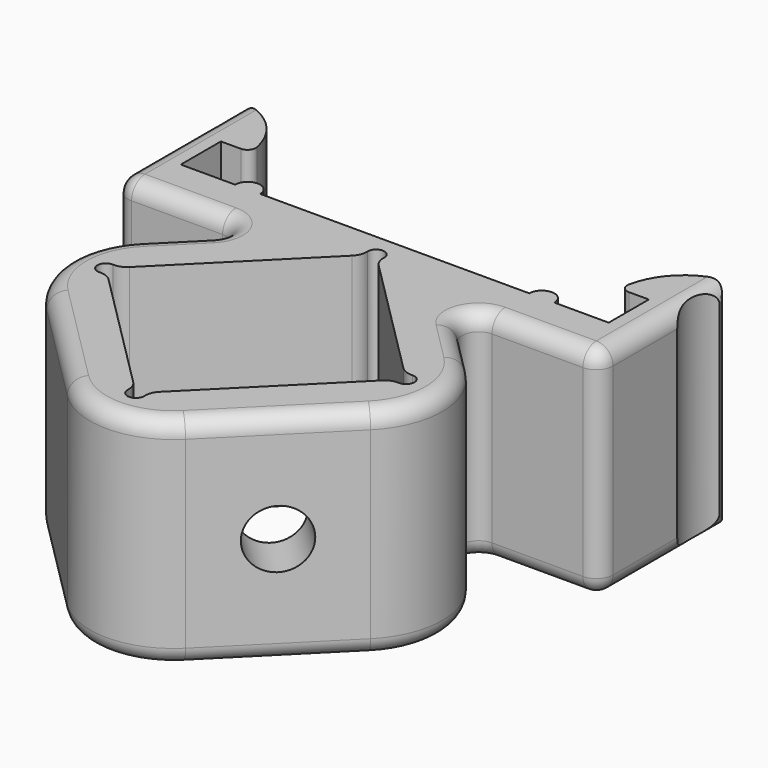
from build123d import *

# Parameters (mm, degrees)
F1_DEPTH  = 13
F4_DEPTH  = 13.001
F5_R      = 0.49999
F6_R      = 1
F7_R      = 5
F8_R      = 1
F9_R      = 0.5
F10_R     = 1
F11_R     = 1.75
F12_DEPTH = 15.6999998824


# Not quite as in the source:
# - a fillet or chamfer is up to 0.001 mm smaller than in the source, because OpenCascade refuses the exact size


with BuildPart() as f1:
    # F0 (on Top) → F1 (new body)
    with BuildSketch(Plane.XY):
        with BuildLine():
            ThreePointArc((-14.5, 1), (-14.2071067812, 0.2928932188), (-13.5, 0))
            Line((-13.5, 0), (-5.6426405208, 0))
            Line((-5.6426405208, 0), (-13.2228966419, -7.5802561211))
            Line((-13.2228966419, -7.5802561211), (0, -20.803152763))
            Line((0, -20.803152763), (13.2228966419, -7.5802561211))
            Line((13.2228966419, -7.5802561211), (5.6426405208, 0))
            Line((5.6426405208, 0), (13.5, 0))
            ThreePointArc((13.5, 0), (14.2071067812, 0.2928932188), (14.5, 1))
            Line((14.5, 1), (14.5, 9.5887489808))
            ThreePointArc((14.5, 9.5887489808), (12.0898455808, 8.3182698074), (11.05, 5.8))
            Line((11.05, 5.8), (12.8, 5.8))
            Line((12.8, 5.8), (12.8, 2.8))
            Line((12.8, 2.8), (9.55, 2.8))
            ThreePointArc((9.55, 2.8), (8.8, 3.55), (8.05, 2.8))
            Line((8.05, 2.8), (-8.05, 2.8))
            ThreePointArc((-8.05, 2.8), (-8.8, 3.55), (-9.55, 2.8))
            Line((-9.55, 2.8), (-12.8, 2.8))
            Line((-12.8, 2.8), (-12.8, 5.8))
            Line((-12.8, 5.8), (-11.05, 5.8))
            ThreePointArc((-11.05, 5.8), (-12.0898455808, 8.3182698074), (-14.5, 9.5887489808))
            Line((-14.5, 9.5887489808), (-14.5, 1))
        make_face()
        with BuildLine():
            Line((-8.6267027305, -7.2267027305), (-0.3535533906, 1.0464466094))
            ThreePointArc((-0.3535533906, 1.0464466094), (0, 1.9), (0.3535533906, 1.0464466094))
            Line((0.3535533906, 1.0464466094), (8.6267027305, -7.2267027305))
            ThreePointArc((8.6267027305, -7.2267027305), (9.4802561211, -7.5802561211), (8.6267027305, -7.9338095117))
            Line((8.6267027305, -7.9338095117), (0.3535533906, -16.2069588515))
            ThreePointArc((0.3535533906, -16.2069588515), (0, -17.0605122421), (-0.3535533906, -16.2069588515))
            Line((-0.3535533906, -16.2069588515), (-8.6267027305, -7.9338095117))
            ThreePointArc((-8.6267027305, -7.9338095117), (-9.4802561211, -7.5802561211), (-8.6267027305, -7.2267027305))
        make_face(mode=Mode.SUBTRACT)
    extrude(amount=F1_DEPTH)

    # F3 (on face) → F4 (cut, through all)
    with BuildSketch(Plane.XY.offset(13)):
        with BuildLine():
            ThreePointArc((-14.5, 5.8), (-14.0485078359, 7.3827532374), (-14.5, 8.9655064748))
            Line((-14.5, 8.9655064748), (-14.5, 5.8))
        make_face()
        with BuildLine():
            Line((14.5, 5.8), (14.5, 8.9655064748))
            ThreePointArc((14.5, 8.9655064748), (14.0485078359, 7.3827532374), (14.5, 5.8))
        make_face()
    extrude(amount=-F4_DEPTH, mode=Mode.SUBTRACT)

    # F5 (radius 0.5 in the source; OpenCascade refuses exactly that, so slightly less here)
    f5_edges = [f1.edges().sort_by_distance(p)[0] for p in [
        (-14.5, 9.588749, 6.5),
        (14.5, 9.588749, 6.5),
    ]]
    fillet(f5_edges, radius=F5_R)

    # F6
    f6_edges = [f1.edges().sort_by_distance(p)[0] for p in [
        (-5.642641, 0, 6.5),
        (5.642641, 0, 6.5),
    ]]
    fillet(f6_edges, radius=F6_R)

    # F7
    f7_edges = [f1.edges().sort_by_distance(p)[0] for p in [
        (-13.222897, -7.580256, 6.5),
        (0, -20.803153, 6.5),
        (13.222897, -7.580256, 6.5),
    ]]
    fillet(f7_edges, radius=F7_R)

    # F8
    f8_edges = [f1.edges().sort_by_distance(p)[0] for p in [
        (-6.611448, -14.191704, 13),
        (-6.611448, -14.191704, 0),
    ]]
    fillet(f8_edges, radius=F8_R)

    # F9
    f9_edges = [f1.edges().sort_by_distance(p)[0] for p in [
        (-11.05, 5.8, 6.5),
        (11.05, 5.8, 6.5),
    ]]
    fillet(f9_edges, radius=F9_R)

    # F10
    f10_edges = [f1.edges().sort_by_distance(p)[0] for p in [
        (-0.353553, 1.046447, 6.5),
        (0.353553, 1.046447, 6.5),
        (-8.626703, -7.226703, 6.5),
        (-8.626703, -7.93381, 6.5),
        (-0.353553, -16.206959, 6.5),
        (0.353553, -16.206959, 6.5),
        (8.626703, -7.226703, 6.5),
        (8.626703, -7.93381, 6.5),
    ]]
    fillet(f10_edges, radius=F10_R)

    # F11 (on face) → F12 (cut, through all)
    with BuildSketch(Plane(origin=(10.4015763815, -10.4015763815, 0), x_dir=(0.7071067812, 0.7071067812, 0), z_dir=(0.7071067812, -0.7071067812, 0))):
        with Locations((-5.3600505063, 6.5)):
            Circle(F11_R)
    extrude(amount=-F12_DEPTH, mode=Mode.SUBTRACT)


solid = f1.part
